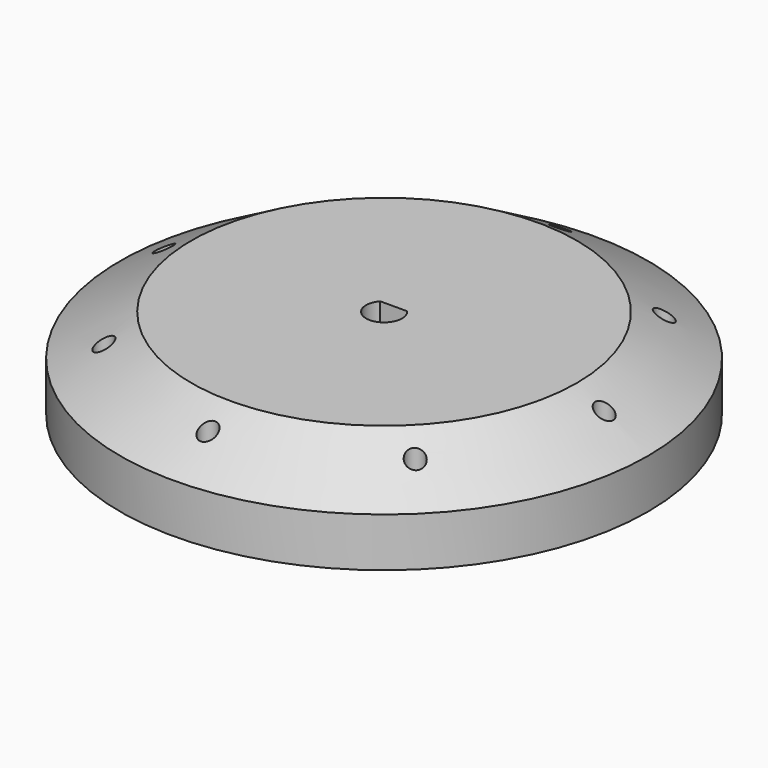
from build123d import *

# Parameters (mm, degrees)
F0_R     = 29.287505
F0_R_2   = 1
F1_DEPTH = 10
F4_W     = 4
F4_H     = 4
F4_R     = 1
F5_DEPTH = 2


# Not quite as in the source:
# - a fillet or chamfer that OpenCascade refuses, or shapes differently, is made with other operations: its cross-section is extruded or revolved along the edge and cut away or added


with BuildPart() as f1:
    # F0 (on Top) → F1 (new body)
    with BuildSketch(Plane.XY):
        Circle(F0_R)
        with Locations((-17.2713695087, -17.2713695087)):
            Circle(F0_R_2, mode=Mode.SUBTRACT)
        with Locations((0, -24.425405)):
            Circle(F0_R_2, mode=Mode.SUBTRACT)
        with Locations((-24.425405, 0)):
            Circle(F0_R_2, mode=Mode.SUBTRACT)
        with BuildLine():
            ThreePointArc((1.4936867141, 1.33), (0, -2), (-1.4936867141, 1.33))
            Line((-1.4936867141, 1.33), (1.4936867141, 1.33))
        make_face(mode=Mode.SUBTRACT)
        with Locations((17.2713695087, -17.2713695087)):
            Circle(F0_R_2, mode=Mode.SUBTRACT)
        with Locations((24.425405, 0)):
            Circle(F0_R_2, mode=Mode.SUBTRACT)
        with Locations((-17.2713695087, 17.2713695087)):
            Circle(F0_R_2, mode=Mode.SUBTRACT)
        with Locations((0, 24.425405)):
            Circle(F0_R_2, mode=Mode.SUBTRACT)
        with Locations((17.2713695087, 17.2713695087)):
            Circle(F0_R_2, mode=Mode.SUBTRACT)
    extrude(amount=F1_DEPTH)

    # F2: chamfer of 7.89245 x 4.55783 on 1 edges, made by hand

    # F2_s1 → F2_t2 (revolve, cut)
    with BuildSketch(Plane.XZ):
        Polygon((29.287505, 5.44217), (21.395055, 10), (29.287505, 10), align=None)
    revolve(axis=Axis((0, 0, 10), (0, 0, 1)), mode=Mode.SUBTRACT)

    # F4 (on offset) → F5 (cut)
    with BuildSketch(Plane.XY.offset(2)):
        with Locations((0, -24.425405)):
            Rectangle(F4_W, F4_H)
        with Locations((0, -24.425405)):
            Circle(F4_R, mode=Mode.SUBTRACT)
        Polygon((-20.0997966335, -17.2713695087), (-17.2713695087, -20.0997966335), (-14.442942384, -17.2713695087), (-17.2713695087, -14.442942384), align=None)
        Polygon((17.2713695087, -20.0997966335), (20.0997966335, -17.2713695087), (17.2713695087, -14.442942384), (14.442942384, -17.2713695087), align=None)
        with Locations((-24.425405, 0)):
            Rectangle(F4_W, F4_H)
        with Locations((24.425405, 0)):
            Rectangle(F4_W, F4_H)
        Polygon((-17.2713695087, 20.0997966335), (-20.0997966335, 17.2713695087), (-17.2713695087, 14.442942384), (-14.442942384, 17.2713695087), align=None)
        Polygon((20.0997966335, 17.2713695087), (17.2713695087, 20.0997966335), (14.442942384, 17.2713695087), (17.2713695087, 14.442942384), align=None)
        with Locations((0, 24.425405)):
            Rectangle(F4_W, F4_H)
        with Locations((0, -24.425405)):
            Circle(F4_R)
    extrude(amount=-F5_DEPTH, mode=Mode.SUBTRACT)


solid = f1.part
